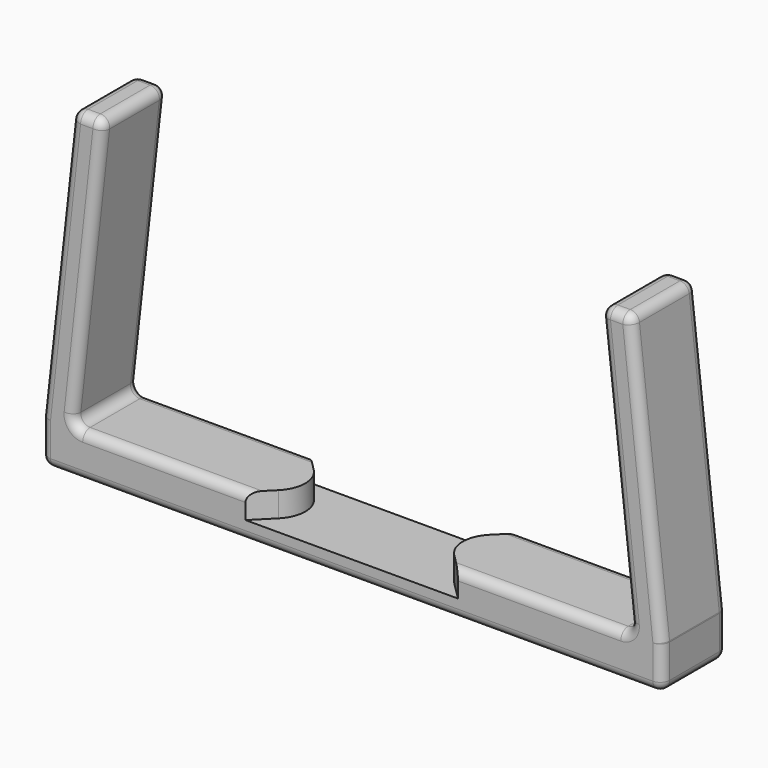
from build123d import *

# Parameters (mm, degrees)
F1_DEPTH = 13
F2_R     = 1.5
F4_DEPTH = 4
F5_ANGLE = -90


with BuildPart() as f1:
    # F0 (on Top) → F1 (new body)
    with BuildSketch(Plane.XY):
        Polygon((-40, -45), (-45, 0), (0, 0), (45, 0), (40, -45), (45, -45), (50, 0), (50, 7), (45, 7), (44.8581193677, 7), (-44.8581193677, 7), (-45, 7), (-50, 7), (-50, 0), (-45, -45), align=None)
    extrude(amount=F1_DEPTH)

    # F2
    f2_edges = [f1.edges().sort_by_distance(p)[0] for p in [
        (-42.5, -22.5, 13),
        (0, 0, 13),
        (42.5, -22.5, 13),
        (42.5, -45, 13),
        (47.5, -22.5, 13),
        (50, 3.5, 13),
        (0, 7, 13),
        (-50, 3.5, 13),
        (-47.5, -22.5, 13),
        (-42.5, -45, 13),
        (-42.5, -22.5, 0),
        (0, 0, 0),
        (42.5, -22.5, 0),
        (42.5, -45, 0),
        (47.5, -22.5, 0),
        (50, 3.5, 0),
        (0, 7, 0),
        (-50, 3.5, 0),
        (-47.5, -22.5, 0),
        (-42.5, -45, 0),
        (40, -45, 6.5),
        (45, -45, 6.5),
        (-45, -45, 6.5),
        (-40, -45, 6.5),
        (-45, 0, 6.5),
        (45, 0, 6.5),
        (-50, 7, 6.5),
        (-50, 0, 6.5),
        (50, 0, 6.5),
        (50, 7, 6.5),
    ]]
    fillet(f2_edges, radius=F2_R)

    # F3 (on face) → F4 (cut)
    with BuildSketch(Plane.XZ):
        with BuildLine():
            Line((-14.1421356237, 2.9644660941), (-15.6066017178, 1.5))
            Line((-15.6066017178, 1.5), (15.6066017178, 1.5))
            Line((15.6066017178, 1.5), (14.1421356237, 2.9644660941))
            ThreePointArc((14.1421356237, 2.9644660941), (12.6776695297, 6.5), (14.1421356237, 10.0355339059))
            Line((14.1421356237, 10.0355339059), (15.6066017178, 11.5))
            Line((15.6066017178, 11.5), (-15.6066017178, 11.5))
            Line((-15.6066017178, 11.5), (-14.1421356237, 10.0355339059))
            ThreePointArc((-14.1421356237, 10.0355339059), (-12.6776695297, 6.5), (-14.1421356237, 2.9644660941))
        make_face()
        Polygon((-24.8033008589, 20.6966991411), (-15.6066017178, 11.5), (15.6066017178, 11.5), (24.8033008589, 20.6966991411), (19.5, 26), (14.1966991411, 31.3033008589), (0, 17.1066017178), (-14.1966991411, 31.3033008589), (-19.5, 26), align=None)
        Polygon((-24.8033008589, -7.6966991411), (-19.5, -13), (-14.1966991411, -18.3033008589), (0, -4.1066017178), (14.1966991411, -18.3033008589), (19.5, -13), (24.8033008589, -7.6966991411), (15.6066017178, 1.5), (-15.6066017178, 1.5), align=None)
    extrude(amount=-F4_DEPTH, mode=Mode.SUBTRACT)


with BuildPart() as f1_1:
    # F5: moved
    add(f1.part.rotate(Axis((0, 4, 0), (1, 0, 0)), F5_ANGLE))


solid = f1_1.part
